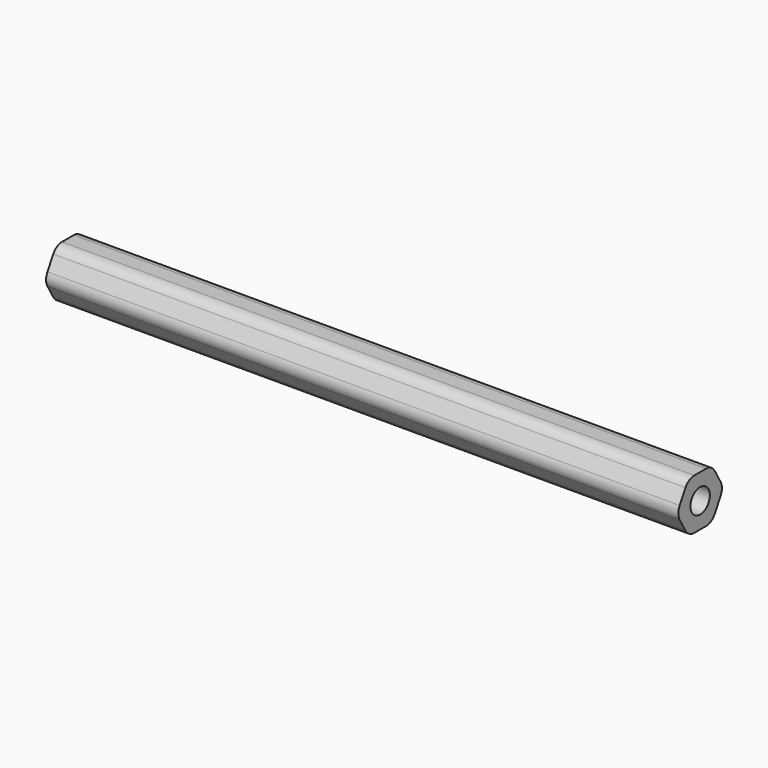
from build123d import *

# Parameters (mm, degrees)
F1_DEPTH = 100
F2_R     = 2
F3_R     = 1.9191209756
F4_DEPTH = 90
F5_R     = 1.25
F6_DEPTH = 20


# Not quite as in the source:
# - a feature names something its author has since deleted; it is built from what else it names


with BuildPart() as f1:
    # F0 (on Right) → F1 (new body)
    with BuildSketch(Plane.YZ):
        Polygon((2.3094010768, 4), (-2.3094010768, 4), (-4.6188021535, 0), (-2.3094010768, -4), (2.3094010768, -4), (4.6188021535, 0), align=None)
    extrude(amount=F1_DEPTH)

    # F2
    f2_edges = [f1.edges().sort_by_distance(p)[0] for p in [
        (50, -2.309401, 4),
        (50, -4.618802, 0),
        (50, -2.309401, -4),
        (50, 2.309401, 4),
        (50, 4.618802, 0),
        (50, 2.309401, -4),
    ]]
    fillet(f2_edges, radius=F2_R)

    # F3 (on face) → F4 (cut)
    with BuildSketch(Plane.YZ.offset(100)):
        Circle(F3_R)
    extrude(amount=-F4_DEPTH, mode=Mode.SUBTRACT)

    # F5 (on face) → F6 (cut)
    with BuildSketch(Plane.YZ.offset(10)):
        Circle(F5_R)
    extrude(amount=-F6_DEPTH, mode=Mode.SUBTRACT)


solid = f1.part
